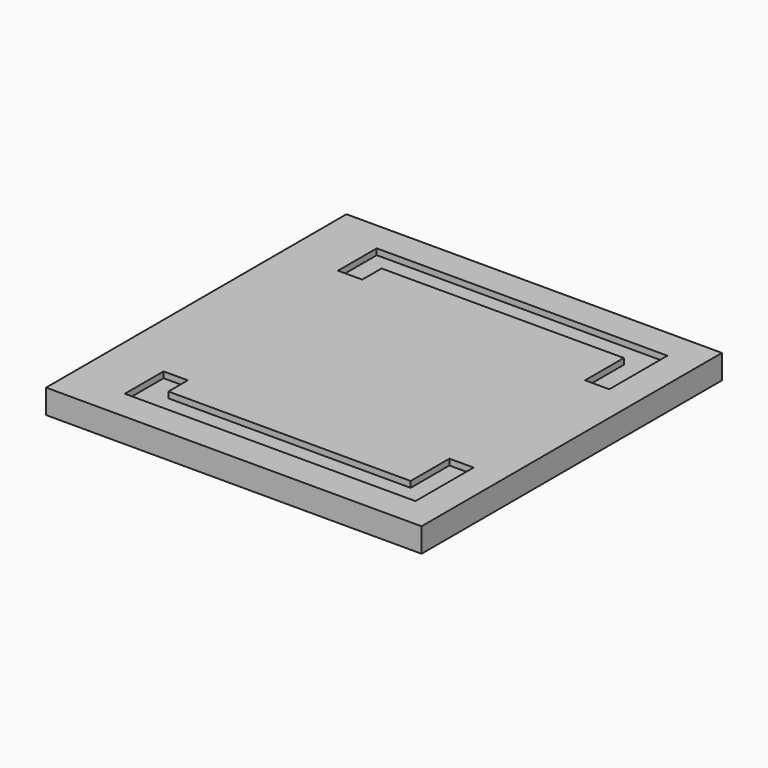
from build123d import *

# Parameters (mm, degrees)
F0_W     = 98.425
F0_H     = 98.425
F1_DEPTH = 3.175
F3_DEPTH = 1.5875


# Not quite as in the source:
# - a pattern or mirror of a feature is missing from the dataset's text; its kind, count and spacing are read off the source's solid


with BuildPart() as f1:
    # F0 (on Top) → F1 (new body, symmetric)
    with BuildSketch(Plane.XY):
        Rectangle(F0_W, F0_H)
    extrude(amount=F1_DEPTH, both=True)

    # F2 (on face) → F3 (cut, symmetric)
    with BuildSketch(Plane.XY.offset(3.175)):
        Polygon((41.275, 22.225), (41.275, 41.275), (-34.925, 41.275), (-34.925, 28.575), (-28.575, 28.575), (-28.575, 34.925), (34.925, 34.925), (34.925, 22.225), align=None)
    f3 = extrude(amount=F3_DEPTH, both=True, mode=Mode.SUBTRACT)

    # F3_copies: F3 across plane
    add(f3.mirror(Plane(origin=(0, 0, 0), x_dir=(0, 0, -1), z_dir=(0, -1, 0))), mode=Mode.SUBTRACT)


solid = f1.part
